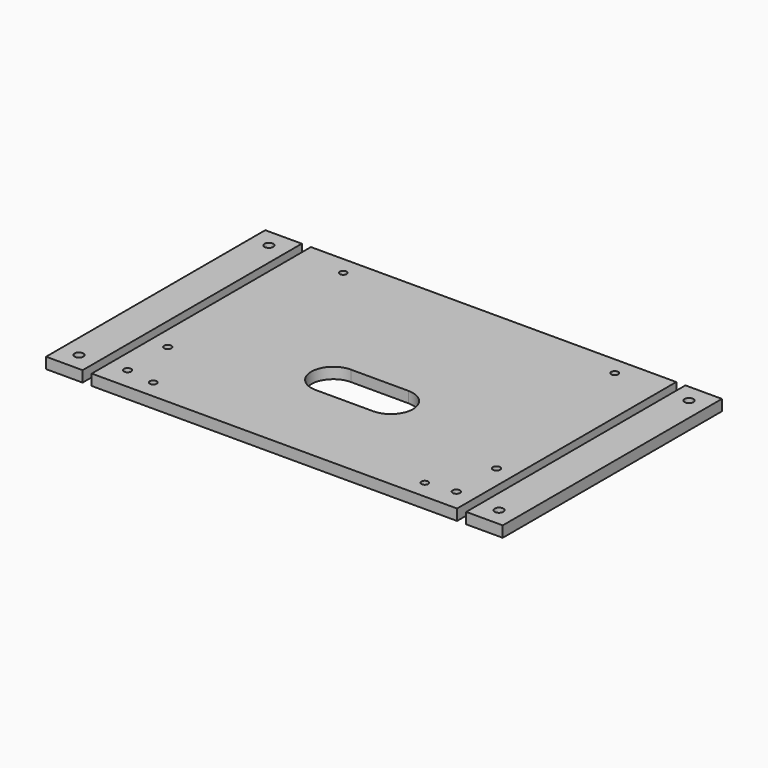
from build123d import *

# Parameters (mm, degrees)
F4_W     = 20
F4_H     = 150
F4_R     = 2.4
F5_DEPTH = 6
F3_W     = 200
F3_H     = 150
F3_R     = 2
F3_R_2   = 1.9


# Not quite as in the source:
# - a pattern or mirror of a feature is missing from the dataset's text; its kind, count and spacing are read off the source's solid
# - a feature names something its author has since deleted; it is built from what else it names


with BuildPart() as f5:
    # F4 (on Top) → F5 (new body)
    with BuildSketch(Plane.XY):
        with Locations((-115, 15)):
            Rectangle(F4_W, F4_H)
        with Locations((-115, -50)):
            Circle(F4_R, mode=Mode.SUBTRACT)
        with Locations((-115, 80)):
            Circle(F4_R, mode=Mode.SUBTRACT)
    extrude(amount=F5_DEPTH)


with BuildPart() as f5b:
    # F3 (on Top) → F5, piece 2 (new body)
    with BuildSketch(Plane.XY):
        with Locations((0, 15)):
            Rectangle(F3_W, F3_H)
        with Locations((-90, -48)):
            Circle(F3_R, mode=Mode.SUBTRACT)
        with Locations((-74.325, -50)):
            Circle(F3_R_2, mode=Mode.SUBTRACT)
        with Locations((-90, -20.5)):
            Circle(F3_R, mode=Mode.SUBTRACT)
        with Locations((74.325, -50)):
            Circle(F3_R_2, mode=Mode.SUBTRACT)
        with Locations((90, -48)):
            Circle(F3_R, mode=Mode.SUBTRACT)
        with BuildLine():
            ThreePointArc((-15.75, -12.075), (-27.825, 0), (-15.75, 12.075))
            Line((-15.75, 12.075), (15.75, 12.075))
            ThreePointArc((15.75, 12.075), (27.825, 0), (15.75, -12.075))
            Line((15.75, -12.075), (-15.75, -12.075))
        make_face(mode=Mode.SUBTRACT)
        with Locations((90, -20.5)):
            Circle(F3_R, mode=Mode.SUBTRACT)
        with Locations((-74.325, 80)):
            Circle(F3_R_2, mode=Mode.SUBTRACT)
        with Locations((74.325, 80)):
            Circle(F3_R_2, mode=Mode.SUBTRACT)
    extrude(amount=F5_DEPTH)


with BuildPart() as f5_copies_1:
    # F5_copies: instance of F5
    add(f5.part.mirror(Plane(origin=(0, 0, 0), x_dir=(0, 0, 1), z_dir=(1, 0, 0))))


solid = Compound([f5.part, f5b.part, f5_copies_1.part])
